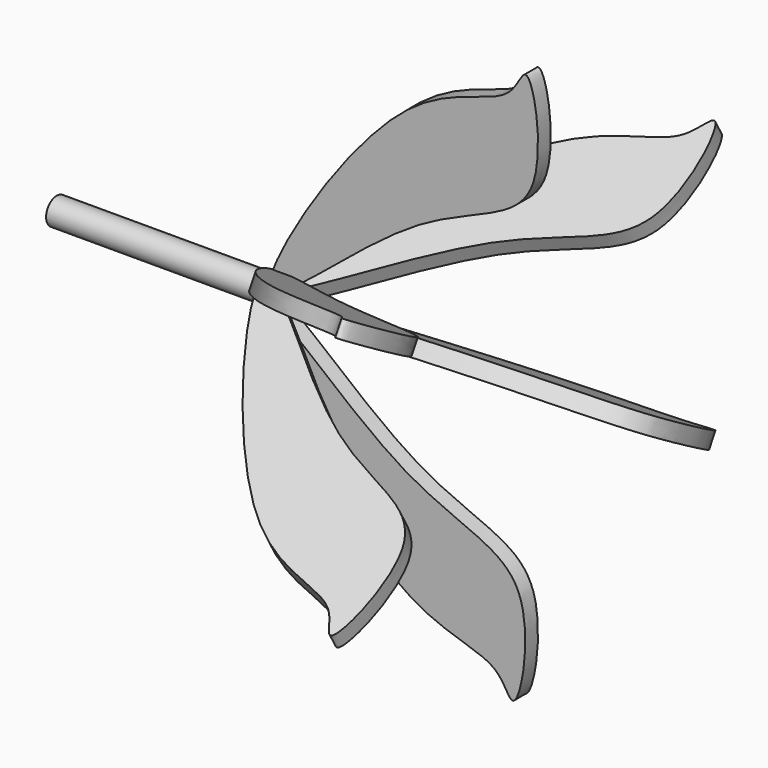
from build123d import *

# Parameters (mm, degrees)
F1_DEPTH = 3
F3_COUNT = 6
F4_W     = 40
F4_H     = 2.5


# Not quite as in the source:
# - the program builds the solid bodies; features that only make, move or delete a surface that nothing else refers to are left out


with BuildPart() as f1:
    # F0 (on Front) → F1 (new body)
    with BuildSketch(Plane.XZ):
        with BuildLine():
            add(Edge.make_bspline(
                [(0, 0), (-1.9268846216, 2.5819970558), (23.3529919407, 45.6267055025), (45.0314889222, 43.7098685189), (48.5023307598, 56.0022828474), (53.6093048303, 26.3962038443), (28.2690449164, 25.5035870387), (1.664508781, -2.230417288), (0, 0)],
                knots=[0, 0, 0, 0, 0.2360644057, 0.3978084995, 0.4740127909, 0.6205229801, 0.7960794996, 1, 1, 1, 1], degree=3))
        make_face()
    extrude(amount=-F1_DEPTH)


with BuildPart() as f3_1:
    # F3: instance of F1
    add(f1.part.rotate(Axis((34.8178520799, 0, 0), (1, 0, 0)), 1 * 360 / F3_COUNT))


with BuildPart() as f3_2:
    # F3: instance of F1
    add(f1.part.rotate(Axis((34.8178520799, 0, 0), (1, 0, 0)), 2 * 360 / F3_COUNT))


with BuildPart() as f3_3:
    # F3: instance of F1
    add(f1.part.rotate(Axis((34.8178520799, 0, 0), (1, 0, 0)), 3 * 360 / F3_COUNT))


with BuildPart() as f3_4:
    # F3: instance of F1
    add(f1.part.rotate(Axis((34.8178520799, 0, 0), (1, 0, 0)), 4 * 360 / F3_COUNT))


with BuildPart() as f3_5:
    # F3: instance of F1
    add(f1.part.rotate(Axis((34.8178520799, 0, 0), (1, 0, 0)), 5 * 360 / F3_COUNT))


with BuildPart() as f5:
    # F4 (on Front) → F5 (revolve)
    with BuildSketch(Plane.XZ):
        with Locations((-20, 1.25)):
            Rectangle(F4_W, F4_H)
    revolve(axis=Axis((-20, 0, 0), (-1, 0, 0)))


solid = Compound([f1.part, f3_1.part, f3_2.part, f3_3.part, f3_4.part, f3_5.part, f5.part])
